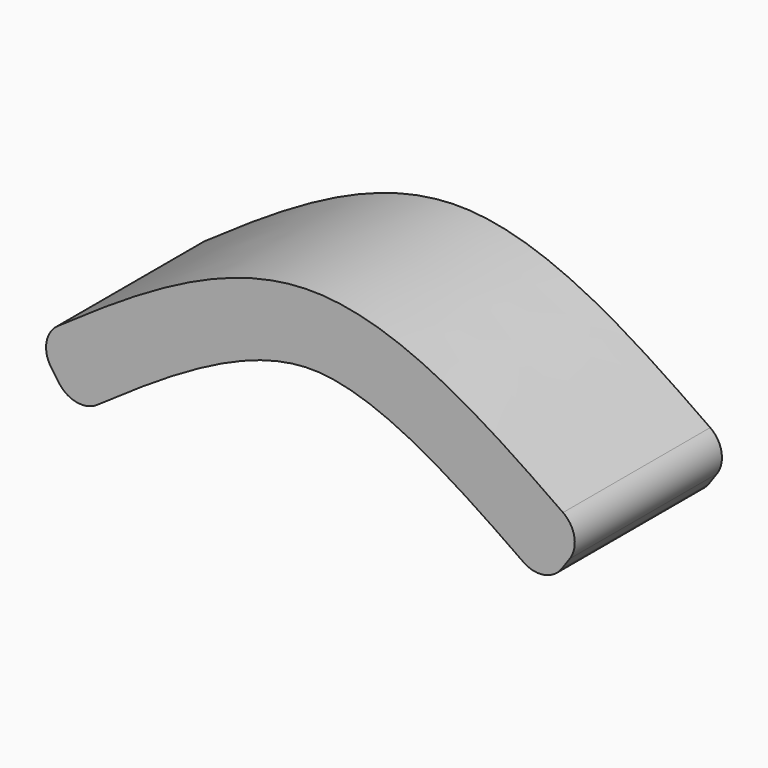
from build123d import *

# Parameters (mm, degrees)
F1_DEPTH = 50.8
F2_R     = 7.62


# Not quite as in the source:
# - the dataset's text gives a spline's control points without its knots; the knots are read off the source's solid


with BuildPart() as f1:
    # F0 (on Front) → F1 (new body)
    with BuildSketch(Plane.XZ):
        with BuildLine():
            add(Edge.make_bspline(
                [(-76.1390706516, -0.0226687638), (-63.4490897984, 8.90261068), (-44.4153157668, 22.2896759075), (-19.0557825534, 33.4461995806), (-0.0516065627, 36.7972034866), (18.9379212805, 33.456137662), (44.2487355385, 22.3000244947), (63.2240707586, 8.9068693117), (75.8750959812, -0.0226420934)],
                knots=[0, 0, 0, 0, 0.25, 0.375, 0.5, 0.625, 0.75, 1, 1, 1, 1], degree=3))
            Line((-76.1390706516, -0.0226687638), (-65.1797871682, -15.6046007856))
            add(Edge.make_bspline(
                [(-65.1797871682, -15.6046007856), (-62.0072930388, -13.3732816869), (-55.7380276393, -8.9643178733), (-46.5724949873, -2.7209730082), (-37.6788903674, 2.9448369362), (-29.1159145991, 7.8332282293), (-22.3268359732, 11.1083959167), (-17.1564484906, 13.1816337612), (-13.4221256972, 14.4532270878), (-9.8419836662, 15.4358831266), (-6.9915610273, 16.014334119), (-4.7889484801, 16.3355540476), (-3.1739749238, 16.5066715187), (-1.8572908328, 16.5918854754), (-0.8188829382, 16.6260233849), (-0.0490443423, 16.634676401), (0.7206704394, 16.6264261107), (1.7585922637, 16.5928391025), (3.0740856825, 16.5083510134), (4.6867686737, 16.3381979335), (6.8852766844, 16.018413363), (9.7288312455, 15.4420456995), (13.2984094164, 14.462303911), (17.0208826474, 13.193639537), (22.174757159, 11.1239255059), (28.942021498, 7.8522008939), (37.4772827137, 2.9662166539), (46.3418125726, -2.6989004591), (55.477608498, -8.943252001), (61.7270611721, -13.3538806664), (64.889793475, -15.5862415758)],
                knots=[0, 0, 0, 0, 0.0625, 0.125, 0.1875, 0.25, 0.3125, 0.34375, 0.375, 0.40625, 0.4375, 0.453125, 0.46875, 0.484375, 0.4921875, 0.5, 0.5078125, 0.515625, 0.53125, 0.546875, 0.5625, 0.59375, 0.625, 0.65625, 0.6875, 0.75, 0.8125, 0.875, 0.9375, 1, 1, 1, 1], degree=3))
            Line((64.889793475, -15.5862415758), (75.8750959812, -0.0226420934))
        make_face()
    extrude(amount=F1_DEPTH)

    # F2
    f2_edges = [f1.edges().sort_by_distance(p)[0] for p in [
        (64.889793, -25.4, -15.586242),
        (75.875096, -25.4, -0.022642),
        (-65.179787, -25.4, -15.604601),
        (-76.139071, -25.4, -0.022669),
    ]]
    fillet(f2_edges, radius=F2_R)


solid = f1.part
